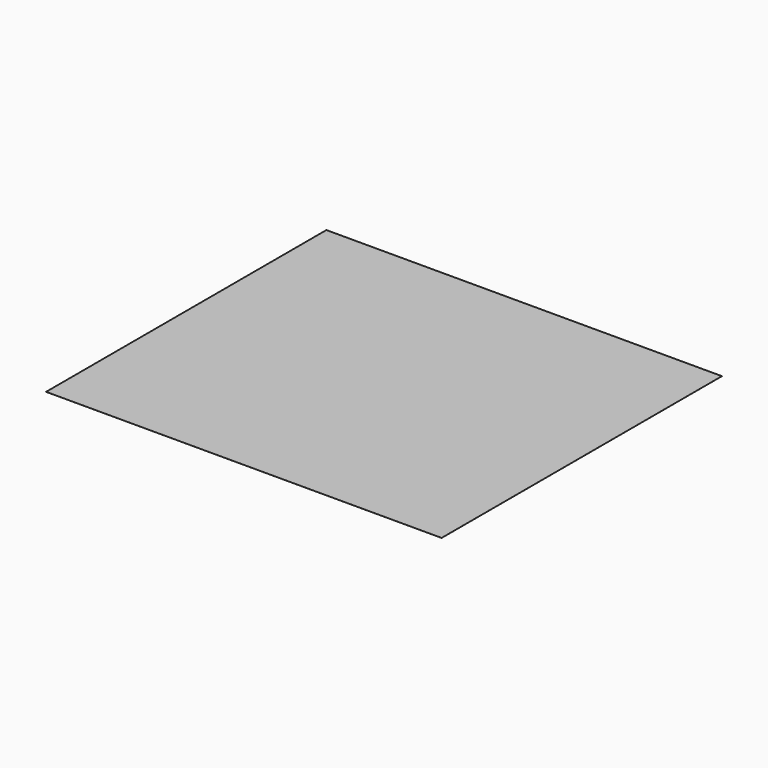
from build123d import *

# Parameters (mm, degrees)
F0_W     = 459.9355608225
F0_H     = 407.4169546366
F1_DEPTH = 0.0254


# Not quite as in the source:
# - the program builds the solid bodies; features that only make, move or delete a surface that nothing else refers to are left out


with BuildPart() as f1:
    # F0 (on Top) → F1 (new body)
    with BuildSketch(Plane.XY):
        with Locations((-203.6788091063, 134.6708461642)):
            Rectangle(F0_W, F0_H)
    extrude(amount=F1_DEPTH)


solid = f1.part
